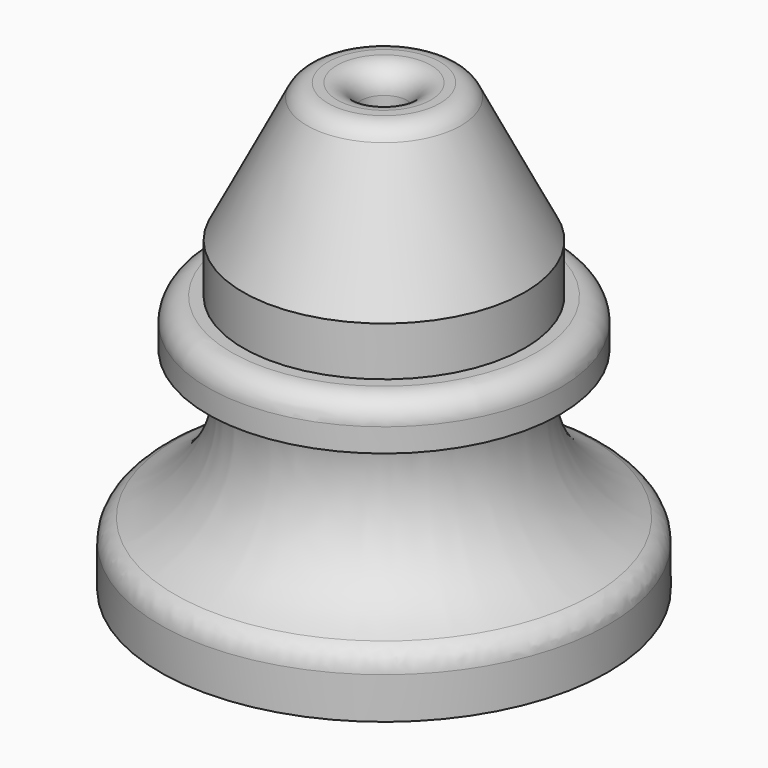
from build123d import *

# Parameters (mm, degrees)
F2_R = 2


with BuildPart() as f1:
    # F0 (on Front) → F1 (revolve)
    with BuildSketch(Plane.XZ):
        with BuildLine():
            Line((6, 23.2861241595), (2, 23.2861241595))
            Line((2, 23.2861241595), (2, 10.2861241595))
            Line((2, 10.2861241595), (9, 10.2861241595))
            ThreePointArc((9, 10.2861241595), (5.8637151227, -4.2318011179), (15.9134753048, -15.1683799922))
            Line((15.9134753048, -15.1683799922), (19.069650506, -14.7138758405))
            Line((19.069650506, -14.7138758405), (19.069650506, -9.7138758405))
            ThreePointArc((19.069650506, -9.7138758405), (12.6596607378, -4.7774457074), (12, 3.2861241595))
            Line((12, 3.2861241595), (15, 3.2861241595))
            Line((15, 3.2861241595), (15, 7.2861241595))
            Line((15, 7.2861241595), (12, 7.2861241595))
            Line((12, 7.2861241595), (12, 11.4697292447))
            Line((12, 11.4697292447), (6, 23.2861241595))
        make_face()
    revolve(axis=Axis((0, 0, 7.4588055012), (0, 0, -1)))

    # F2
    f2_edges = [f1.edges().sort_by_distance(p)[0] for p in [
        (-15, 0, 7.286124),
        (-19.069651, 0, -9.713876),
        (-6, 0, 23.286124),
        (-2, 0, 23.286124),
    ]]
    fillet(f2_edges, radius=F2_R)


solid = f1.part
